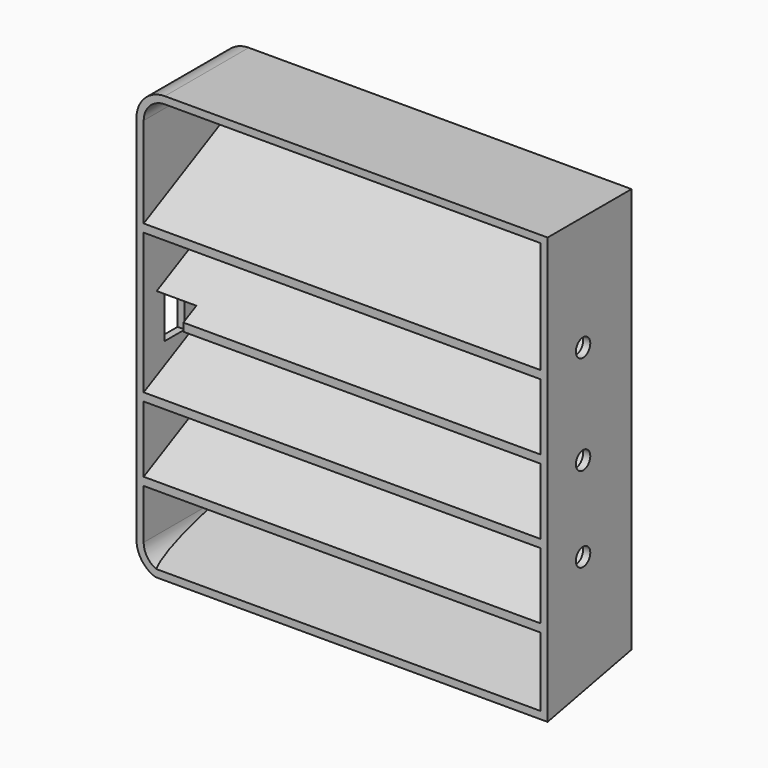
from build123d import *

# Parameters (mm, degrees)
F1_DEPTH    = 37
F2_T1_DEPTH = 342.8505669038
F3_T        = -2.54
F4_W        = 125.55387271
F4_H        = 111.9176980871
F5_DEPTH    = 25.4
F6_R        = 3.175
F7_DEPTH    = 19.05
F9_DEPTH    = 142.24
F10_W       = 9
F10_H       = 17.5
F11_DEPTH   = 16.5
F13_DEPTH   = 14


# Not quite as in the source:
# - a fillet or chamfer that OpenCascade refuses, or shapes differently, is made with other operations: its cross-section is extruded or revolved along the edge and cut away or added
# - a feature names something its author has since deleted; it is built from what else it names


with BuildPart() as f1:
    # F0 (on Front) → F1 (new body)
    with BuildSketch(Plane.XZ):
        with BuildLine():
            Line((72.5, 75.5), (-62.5, 75.5))
            ThreePointArc((-62.5, 75.5), (-69.5710678119, 72.5710678119), (-72.5, 65.5))
            Line((-72.5, 65.5), (-72.5, -65.5))
            ThreePointArc((-72.5, -65.5), (-69.5710678119, -72.5710678119), (-62.5, -75.5))
            Line((-62.5, -75.5), (72.5, -75.5))
            Line((72.5, -75.5), (72.5, 75.5))
        make_face()
    extrude(amount=F1_DEPTH)

    # F2: chamfer of 40 x 8 on 1 edges, made by hand

    # F2_s2 → F2_t1 (cut)
    with BuildSketch(Plane.YZ.offset(-166.4252834519)):
        Polygon((-40, -75.5), (0, -67.5), (0, -75.5), align=None)
    extrude(amount=F2_T1_DEPTH, mode=Mode.SUBTRACT)

    # F3
    f3_openings = [f1.faces().sort_by_distance(p)[0] for p in [
        (0.123954, -37, 0.284541),
    ]]
    offset(amount=F3_T, openings=f3_openings)

    # F4 (on face) → F5 (cut)
    with BuildSketch(Plane.XZ.offset(2.54)):
        with Locations((-0.276936355, 9.5411509565)):
            Rectangle(F4_W, F4_H)
    extrude(amount=-F5_DEPTH, mode=Mode.SUBTRACT)

    # F6 (on face) → F7 (cut)
    with BuildSketch(Plane(origin=(69.96, 0, 0), x_dir=(0, -1, 0), z_dir=(-1, 0, 0))):
        with Locations((21.3561020792, 0)):
            Circle(F6_R)
        with Locations((21.3561020792, 35)):
            Circle(F6_R)
        with Locations((21.3561020792, -30)):
            Circle(F6_R)
    extrude(amount=-F7_DEPTH, mode=Mode.SUBTRACT)

    # F8 (on face) → F9 (join)
    with BuildSketch(Plane(origin=(69.96, 0, 0), x_dir=(0, -1, 0), z_dir=(-1, 0, 0))):
        Polygon((0, -29.2355429628), (37, -47.9510980871), (37, -45.1046433113), (0, -26.389088187), align=None)
        Polygon((0, -3.021088187), (37, -21.7366433113), (37, -18.8901885355), (0, -0.1746334112), align=None)
        Polygon((0, 23.1933665888), (37, 4.4778114645), (37, 7.3242662403), (0, 26.0398213646), align=None)
        Polygon((0, 49.4078213646), (37, 30.6922662403), (37, 33.5387210161), (0, 52.2542761405), align=None)
    extrude(amount=F9_DEPTH)

    # F10 (on face) → F11 (cut)
    with BuildSketch(Plane(origin=(-72.5, 0, 0), x_dir=(0, -1, 0), z_dir=(-1, 0, 0))):
        with Locations((23.4, 2)):
            Rectangle(F10_W, F10_H)
    extrude(amount=-F11_DEPTH, mode=Mode.SUBTRACT)

    # F12 (on face) → F13 (cut)
    with BuildSketch(Plane.YZ.offset(-69.96)):
        Polygon((-44.6556091905, -6.75), (-37, -6.75), (-37, 4.4778114645), (-27.9, 9.0808263735), (-27.9, 10.2238561958), (-44.6556091905, 10.2238561958), align=None)
    extrude(amount=F13_DEPTH, mode=Mode.SUBTRACT)


solid = f1.part
